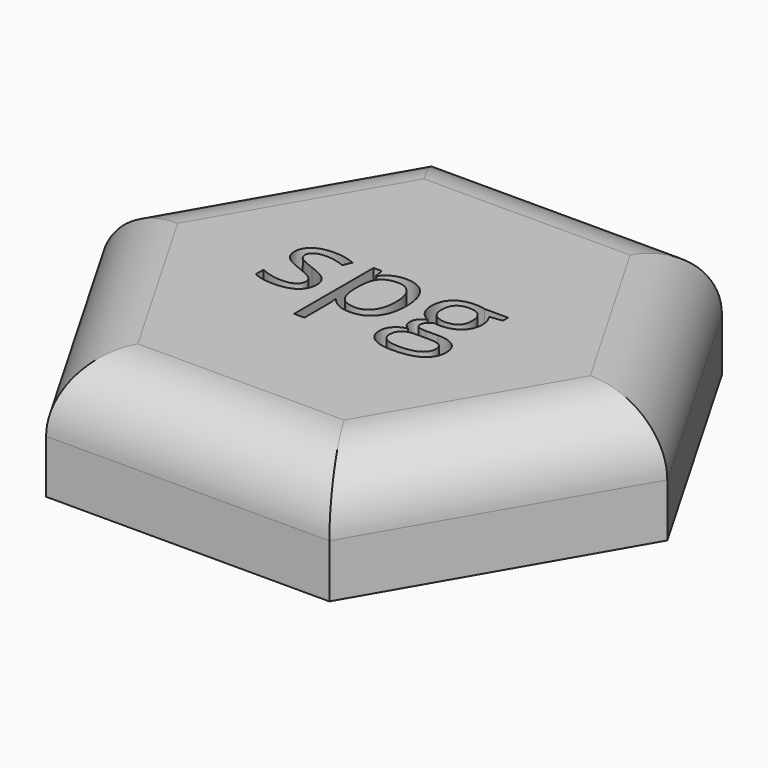
from build123d import *

# Parameters (mm, degrees)
F1_DEPTH     = 99
F2_R         = 55
F3_TEXT_SIZE = 105.6328829792
F4_DEPTH     = 99.001


# Not quite as in the source:
# - Text() gives the source's letters only with a copy of the font that has no kerning and outlines rounded to 1/6400 em; it was checked with that copy


with BuildPart() as f1:
    # F0 (on Top) → F1 (new body)
    with BuildSketch(Plane.XY):
        Polygon((-116.8454818649, 0), (116.8454818649, 0), (233.6909637299, 202.3823112249), (116.8454818649, 404.7646224499), (-116.8454818649, 404.7646224499), (-233.6909637299, 202.3823112249), align=None)
    extrude(amount=F1_DEPTH)

    # F2
    f2_edges = [f1.edges().sort_by_distance(p)[0] for p in [
        (-175.268223, 101.191156, 99),
        (0, 0, 99),
        (175.268223, 101.191156, 99),
        (175.268223, 303.573467, 99),
        (0, 404.764622, 99),
        (-175.268223, 303.573467, 99),
    ]]
    fillet(f2_edges, radius=F2_R)

    # F3 (on face) → F4 (cut, through all)
    with BuildSketch(Plane.XY.offset(99)):
        with Locations((-92.2234801038, 175.9981513023)):
            Text('spg', F3_TEXT_SIZE, font='Open Sans', text_align=(TextAlign.LEFT, TextAlign.BOTTOM))
    extrude(amount=-F4_DEPTH, mode=Mode.SUBTRACT)


solid = f1.part
